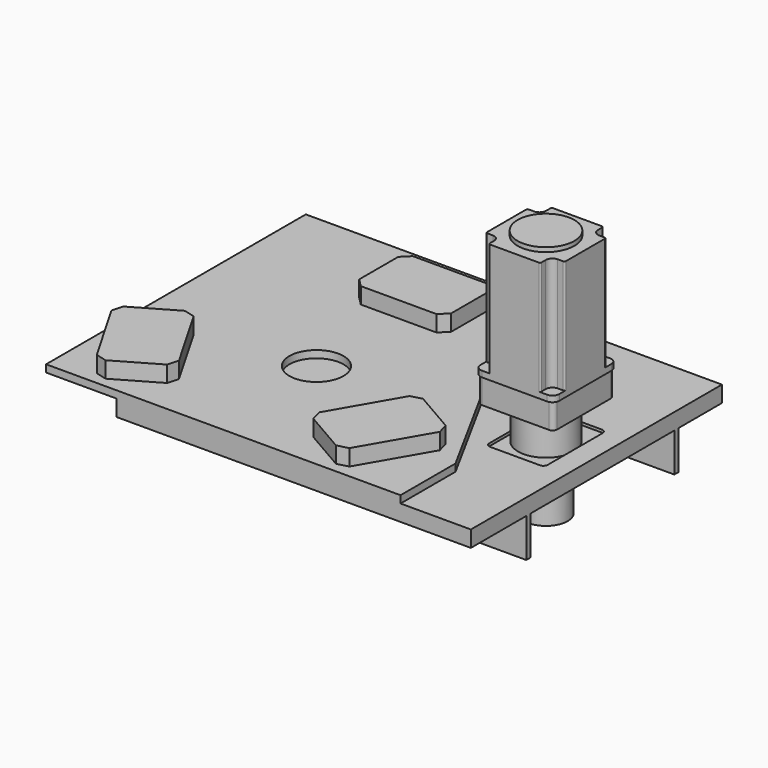
from build123d import *

# Parameters (mm, degrees)
F0_W         = 655
F0_H         = 30
F1_DEPTH     = 580
F3_DEPTH     = 13.5
F5_DEPTH     = 5
F6_R         = 51.5
F7_DEPTH     = 67
F9_DEPTH     = 47
F11_DEPTH    = 11
F13_DEPTH    = 210
F14_R        = 52.5
F15_DEPTH    = 8
F16_R        = 50
F17_DEPTH    = 13.5
F18_W        = 170
F18_H        = 120
F19_DEPTH    = 30
F20_SIZE     = 15
F21_T1_DEPTH = 68.5752448195
F22_W        = 655
F22_H        = 10
F23_DEPTH    = 71.7
F24_R        = 25
F25_DEPTH    = 42
F26_R        = 40
F27_DEPTH    = 50


# Not quite as in the source:
# - a fillet or chamfer that OpenCascade refuses, or shapes differently, is made with other operations: its cross-section is extruded or revolved along the edge and cut away or added


with BuildPart() as f1:
    # F0 (on Front) → F1 (new body)
    with BuildSketch(Plane.XZ):
        with Locations((35.6008394094, 15)):
            Rectangle(F0_W, F0_H)
    extrude(amount=F1_DEPTH)

    # F2 (on face) → F3 (join)
    with BuildSketch(Plane.XY.offset(30)):
        Polygon((-422.0060110092, -580), (233.1008394094, -580), (233.1008394094, -453), (-25.8483879637, 20), (-422.0060110092, 20), align=None)
    extrude(amount=F3_DEPTH)

    # F4 (on face) → F5 (cut)
    with BuildSketch(Plane.XY.offset(30)):
        with BuildLine():
            Line((315.5072791576, -218), (223.5072791576, -218))
            ThreePointArc((223.5072791576, -218), (217.8504249081, -220.3431457505), (215.5072791576, -226))
            Line((215.5072791576, -226), (215.5072791576, -353))
            ThreePointArc((215.5072791576, -353), (217.8504249081, -358.6568542495), (223.5072791576, -361))
            Line((223.5072791576, -361), (315.5072791576, -361))
            ThreePointArc((315.5072791576, -361), (321.1641334071, -358.6568542495), (323.5072791576, -353))
            Line((323.5072791576, -353), (323.5072791576, -226))
            ThreePointArc((323.5072791576, -226), (321.1641334071, -220.3431457505), (315.5072791576, -218))
        make_face()
    extrude(amount=-F5_DEPTH, mode=Mode.SUBTRACT)

    # F6 (on face) → F7 (join)
    with BuildSketch(Plane.XY.offset(25)):
        with Locations((269.5072791576, -289.5)):
            Circle(F6_R)
    extrude(amount=F7_DEPTH)

    # F8 (on face) → F9 (join)
    with BuildSketch(Plane.XY.offset(92)):
        with BuildLine():
            Line((331.5072791576, -219.5), (207.5072791576, -219.5))
            ThreePointArc((207.5072791576, -219.5), (201.8504249081, -221.8431457505), (199.5072791576, -227.5))
            Line((199.5072791576, -227.5), (199.5072791576, -351.5))
            ThreePointArc((199.5072791576, -351.5), (201.8504249081, -357.1568542495), (207.5072791576, -359.5))
            Line((207.5072791576, -359.5), (331.5072791576, -359.5))
            ThreePointArc((331.5072791576, -359.5), (337.1641334071, -357.1568542495), (339.5072791576, -351.5))
            Line((339.5072791576, -351.5), (339.5072791576, -227.5))
            ThreePointArc((339.5072791576, -227.5), (337.1641334071, -221.8431457505), (331.5072791576, -219.5))
        make_face()
    extrude(amount=F9_DEPTH)

    # F10 (on face) → F11 (join)
    with BuildSketch(Plane.XY.offset(139)):
        with BuildLine():
            Line((329.8072791576, -216.7), (209.2072791576, -216.7))
            ThreePointArc((209.2072791576, -216.7), (200.3684443928, -220.3611652352), (196.7072791576, -229.2))
            Line((196.7072791576, -229.2), (196.7072791576, -349.8))
            ThreePointArc((196.7072791576, -349.8), (200.3684443928, -358.6388347648), (209.2072791576, -362.3))
            Line((209.2072791576, -362.3), (329.8072791576, -362.3))
            ThreePointArc((329.8072791576, -362.3), (338.6461139225, -358.6388347648), (342.3072791576, -349.8))
            Line((342.3072791576, -349.8), (342.3072791576, -229.2))
            ThreePointArc((342.3072791576, -229.2), (338.6461139225, -220.3611652352), (329.8072791576, -216.7))
        make_face()
    extrude(amount=F11_DEPTH)

    # F12 (on face) → F13 (join)
    with BuildSketch(Plane.XY.offset(150)):
        with BuildLine():
            ThreePointArc((221.6497197978, -359.5550261631), (222.4537040204, -361.4960157773), (224.3946936347, -362.3))
            Line((224.3946936347, -362.3), (314.5623053207, -362.3))
            ThreePointArc((314.5623053207, -362.3), (316.503294935, -361.4960157773), (317.3072791576, -359.5550261631))
            Line((317.3072791576, -359.5550261631), (317.3072791576, -349.8))
            ThreePointArc((317.3072791576, -349.8), (320.7925325094, -341.1406499743), (329.3047740164, -337.3101045407))
            ThreePointArc((329.3047740164, -337.3101045407), (329.8072791576, -337.3), (330.3097842989, -337.3101045407))
            Line((330.3097842989, -337.3101045407), (339.5623053207, -337.3101045407))
            ThreePointArc((339.5623053207, -337.3101045407), (341.503294935, -336.5061203181), (342.3072791576, -334.5651307038))
            Line((342.3072791576, -334.5651307038), (342.3072791576, -244.4433875239))
            ThreePointArc((342.3072791576, -244.4433875239), (341.503294935, -242.5023979096), (339.5623053207, -241.698413687))
            Line((339.5623053207, -241.698413687), (330.006415567, -241.698413687))
            ThreePointArc((330.006415567, -241.698413687), (321.7732212328, -238.7762160199), (317.4644895357, -231.1762450125))
            ThreePointArc((317.4644895357, -231.1762450125), (317.3072791576, -229.2), (317.4644895357, -227.2237549875))
            Line((317.4644895357, -227.2237549875), (317.4644895357, -219.4449738369))
            ThreePointArc((317.4644895357, -219.4449738369), (316.6605053131, -217.5039842227), (314.7195156988, -216.7))
            Line((314.7195156988, -216.7), (224.4374317064, -216.7))
            ThreePointArc((224.4374317064, -216.7), (222.4949663799, -217.5054610577), (221.6924610453, -219.4491493681))
            Line((221.6924610453, -219.4491493681), (221.7072646957, -229.18098556))
            ThreePointArc((221.7072646957, -229.18098556), (218.1514308097, -237.9322477762), (209.4879256393, -241.696849105))
            ThreePointArc((209.4879256393, -241.696849105), (209.2072791576, -241.7), (208.926632676, -241.696849105))
            Line((208.926632676, -241.696849105), (199.4522529946, -241.696849105))
            ThreePointArc((199.4522529946, -241.696849105), (197.5112633803, -242.5008333276), (196.7072791576, -244.4418229419))
            Line((196.7072791576, -244.4418229419), (196.7072791576, -334.5586429094))
            ThreePointArc((196.7072791576, -334.5586429094), (197.5112633803, -336.4996325237), (199.4522529946, -337.3036167464))
            Line((199.4522529946, -337.3036167464), (208.906603954, -337.3036167464))
            ThreePointArc((208.906603954, -337.3036167464), (209.2072791576, -337.3), (209.5079543613, -337.3036167464))
            ThreePointArc((209.5079543613, -337.3036167464), (217.722501739, -340.6489899798), (221.6497197978, -348.6018051423))
            ThreePointArc((221.6497197978, -348.6018051423), (221.7072791576, -349.8), (221.6497197978, -350.9981948577))
            Line((221.6497197978, -350.9981948577), (221.6497197978, -359.5550261631))
        make_face()
        with BuildLine():
            Line((221.6497197978, -348.6018051423), (221.6497197978, -350.9981948577))
            ThreePointArc((221.6497197978, -350.9981948577), (221.7072791576, -349.8), (221.6497197978, -348.6018051423))
        make_face()
        with BuildLine():
            ThreePointArc((330.3097842989, -337.3101045407), (329.8072791576, -337.3), (329.3047740164, -337.3101045407))
            Line((329.3047740164, -337.3101045407), (330.3097842989, -337.3101045407))
        make_face()
        with BuildLine():
            Line((208.906603954, -337.3036167464), (209.5079543613, -337.3036167464))
            ThreePointArc((209.5079543613, -337.3036167464), (209.2072791576, -337.3), (208.906603954, -337.3036167464))
        make_face()
        with BuildLine():
            Line((209.4879256393, -241.696849105), (208.926632676, -241.696849105))
            ThreePointArc((208.926632676, -241.696849105), (209.2072791576, -241.7), (209.4879256393, -241.696849105))
        make_face()
        with BuildLine():
            ThreePointArc((317.4644895357, -227.2237549875), (317.3072791576, -229.2), (317.4644895357, -231.1762450125))
            Line((317.4644895357, -231.1762450125), (317.4644895357, -227.2237549875))
        make_face()
    extrude(amount=F13_DEPTH)

    # F14 (on face) → F15 (join)
    with BuildSketch(Plane.XY.offset(360)):
        with Locations((269.5072791576, -289.5)):
            Circle(F14_R)
    extrude(amount=F15_DEPTH)

    # F16 (on face) → F17 (cut)
    with BuildSketch(Plane.XY.offset(43.5)):
        with Locations((-113.8991605906, -340.5)):
            Circle(F16_R)
    extrude(amount=-F17_DEPTH, mode=Mode.SUBTRACT)

    # F18 (on face) → F19 (join)
    with BuildSketch(Plane.XY.offset(43.5)):
        with Locations((-113.8991605906, -90.5)):
            Rectangle(F18_W, F18_H)
        Polygon((-424.8670357638, -421.8878406783), (-339.8670357638, -569.1121593217), (-235.9439873097, -509.1121593217), (-320.9439873097, -361.8878406783), align=None)
        Polygon((112.0687145825, -569.1121593217), (197.0687145825, -421.8878406783), (93.1456661284, -361.8878406783), (8.1456661284, -509.1121593217), align=None)
    extrude(amount=F19_DEPTH)

    # F20
    f20_edges = [f1.edges().sort_by_distance(p)[0] for p in [
        (-198.899161, -30.5, 58.5),
    ]]
    chamfer(f20_edges, length=F20_SIZE)

    # F21: chamfer of 15 on 11 edges, made by hand

    # F21_s2 → F21_t1 (cut)
    with BuildSketch(Plane.XY.offset(43.5)):
        Polygon((-43.8991605906, -30.5), (-28.8991605906, -45.5), (-28.8991605906, -30.5), align=None)
        Polygon((106.1360471852, -369.3878406783), (85.6456661284, -374.8782217351), (93.1456661284, -361.8878406783), align=None)
        Polygon((15.6456661284, -496.1217782649), (21.1360471852, -516.6121593217), (8.1456661284, -509.1121593217), align=None)
        Polygon((119.5687145825, -556.1217782649), (99.0783335258, -561.6121593217), (112.0687145825, -569.1121593217), align=None)
        Polygon((189.5687145825, -434.8782217351), (184.0783335258, -414.3878406783), (197.0687145825, -421.8878406783), align=None)
        Polygon((-28.8991605906, -135.5), (-43.8991605906, -150.5), (-28.8991605906, -150.5), align=None)
        Polygon((-198.8991605906, -135.5), (-183.8991605906, -150.5), (-198.8991605906, -150.5), align=None)
        Polygon((-248.9343683664, -516.6121593217), (-243.4439873097, -496.1217782649), (-235.9439873097, -509.1121593217), align=None)
        Polygon((-347.3670357638, -556.1217782649), (-326.876654707, -561.6121593217), (-339.8670357638, -569.1121593217), align=None)
        Polygon((-417.3670357638, -434.8782217351), (-411.876654707, -414.3878406783), (-424.8670357638, -421.8878406783), align=None)
        Polygon((-313.4439873097, -374.8782217351), (-333.9343683664, -369.3878406783), (-320.9439873097, -361.8878406783), align=None)
    extrude(amount=F21_T1_DEPTH, mode=Mode.SUBTRACT)

    # F22 (on face) → F23 (join)
    with BuildSketch(Plane(origin=(0, 0, 0), x_dir=(1, 0, 0), z_dir=(0, 0, -1))):
        with Locations((35.6008394094, 105)):
            Rectangle(F22_W, F22_H)
        with Locations((35.6008394094, 447)):
            Rectangle(F22_W, F22_H)
    extrude(amount=F23_DEPTH)

    # F24 (on face) → F25 (join)
    with BuildSketch(Plane(origin=(0, 0, 0), x_dir=(1, 0, 0), z_dir=(0, 0, -1))):
        with Locations((269.5072791576, 289.5)):
            Circle(F24_R)
    extrude(amount=F25_DEPTH)

    # F26 (on face) → F27 (join)
    with BuildSketch(Plane(origin=(0, 0, -42), x_dir=(1, 0, 0), z_dir=(0, 0, -1))):
        with Locations((269.5072791576, 289.5)):
            Circle(F26_R)
    extrude(amount=F27_DEPTH)


solid = f1.part
